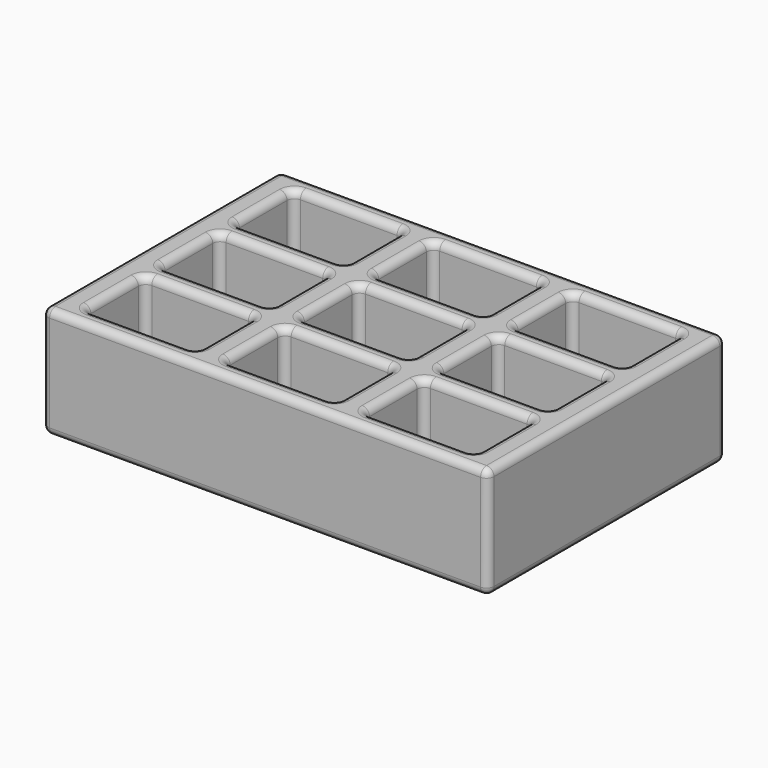
from build123d import *

# Parameters (mm, degrees)
F0_W     = 120
F0_H     = 80
F1_DEPTH = 30
F2_W     = 30
F2_H     = 20
F3_DEPTH = 20
F4_R     = 2


with BuildPart() as f1:
    # F0 (on Top) → F1 (new body)
    with BuildSketch(Plane.XY):
        Rectangle(F0_W, F0_H)
    extrude(amount=F1_DEPTH)

    # F2 (on face) → F3 (cut)
    with BuildSketch(Plane.XY.offset(30)):
        with Locations((-37.5, 25)):
            Rectangle(F2_W, F2_H)
        with Locations((0, 25)):
            Rectangle(F2_W, F2_H)
        with Locations((37.5, 25)):
            Rectangle(F2_W, F2_H)
        with Locations((37.5, 0)):
            Rectangle(F2_W, F2_H)
        Rectangle(F2_W, F2_H)
        with Locations((-37.5, 0)):
            Rectangle(F2_W, F2_H)
        with Locations((-37.5, -25)):
            Rectangle(F2_W, F2_H)
        with Locations((0, -25)):
            Rectangle(F2_W, F2_H)
        with Locations((37.5, -25)):
            Rectangle(F2_W, F2_H)
    extrude(amount=-F3_DEPTH, mode=Mode.SUBTRACT)

    # F4
    f4_edges = [f1.edges().sort_by_distance(p)[0] for p in [
        (-37.5, 35, 10),
        (-52.5, 25, 10),
        (-37.5, 15, 10),
        (-22.5, 25, 10),
        (-52.5, 35, 20),
        (-52.5, 15, 20),
        (-52.5, 25, 30),
        (-22.5, 35, 20),
        (-37.5, 35, 30),
        (-22.5, 15, 20),
        (-37.5, 15, 30),
        (-22.5, 25, 30),
        (-15, 35, 20),
        (-15, 15, 20),
        (-15, 25, 30),
        (-15, 25, 10),
        (15, 15, 20),
        (15, 35, 20),
        (15, 25, 30),
        (15, 25, 10),
        (22.5, 35, 20),
        (22.5, 15, 20),
        (22.5, 25, 30),
        (22.5, 25, 10),
        (52.5, 15, 20),
        (52.5, 35, 20),
        (52.5, 25, 30),
        (52.5, 25, 10),
        (-22.5, -10, 20),
        (-22.5, 10, 20),
        (-22.5, 0, 30),
        (-22.5, 0, 10),
        (15, -35, 20),
        (15, -15, 20),
        (15, -25, 30),
        (15, -25, 10),
        (15, -10, 20),
        (15, 10, 20),
        (15, 0, 30),
        (15, 0, 10),
        (-15, -10, 20),
        (0, -10, 30),
        (0, -10, 10),
        (-15, 10, 20),
        (-15, 0, 30),
        (-15, 0, 10),
        (-52.5, 10, 20),
        (-52.5, -10, 20),
        (-52.5, 0, 30),
        (-52.5, 0, 10),
        (-52.5, -15, 20),
        (-52.5, -35, 20),
        (-52.5, -25, 30),
        (-52.5, -25, 10),
        (-15, -15, 20),
        (-15, -35, 20),
        (-15, -25, 30),
        (-15, -25, 10),
        (22.5, -15, 20),
        (22.5, -35, 20),
        (22.5, -25, 30),
        (22.5, -25, 10),
        (22.5, 10, 20),
        (22.5, -10, 20),
        (22.5, 0, 30),
        (22.5, 0, 10),
        (52.5, -15, 20),
        (37.5, -15, 30),
        (37.5, -15, 10),
        (52.5, -35, 20),
        (52.5, -25, 30),
        (52.5, -25, 10),
        (52.5, -10, 20),
        (52.5, 10, 20),
        (52.5, 0, 30),
        (52.5, 0, 10),
        (-22.5, -35, 20),
        (-22.5, -15, 20),
        (-22.5, -25, 30),
        (-22.5, -25, 10),
        (-60, 40, 15),
        (-60, -40, 15),
        (60, -40, 15),
        (0, -40, 0),
        (0, -40, 30),
        (60, 40, 15),
        (60, 0, 0),
        (60, 0, 30),
        (-60, 0, 0),
        (-60, 0, 30),
        (0, 40, 0),
        (0, 40, 30),
        (-37.5, -15, 30),
        (-37.5, -35, 30),
        (0, -15, 30),
        (0, -35, 30),
        (37.5, -35, 30),
        (-37.5, 10, 30),
        (-37.5, -10, 30),
        (0, 10, 30),
        (37.5, -10, 30),
        (37.5, 10, 30),
        (0, 35, 30),
        (0, 15, 30),
        (37.5, 35, 30),
        (37.5, 15, 30),
    ]]
    fillet(f4_edges, radius=F4_R)


solid = f1.part
